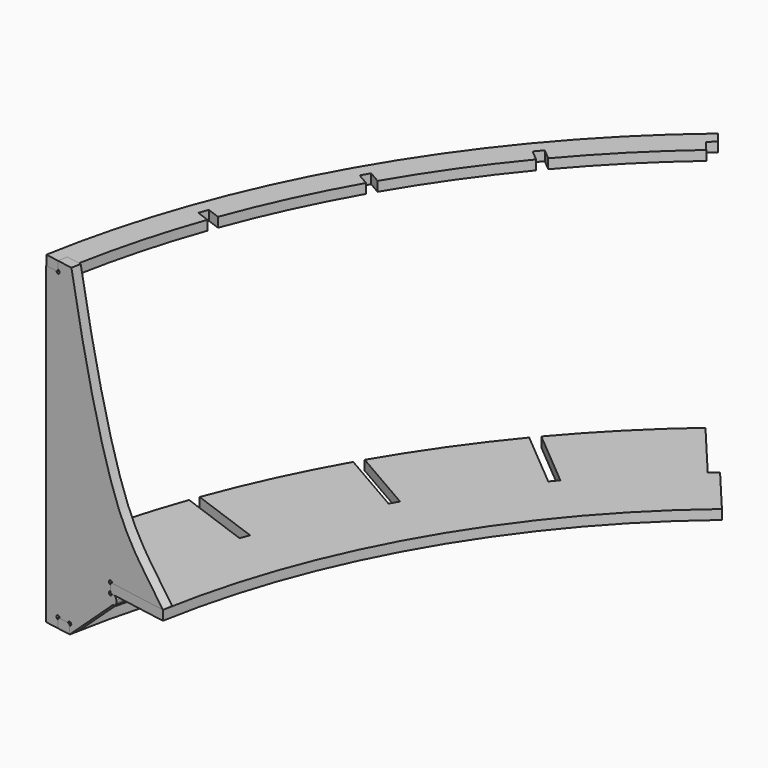
from build123d import *

# Parameters (mm, degrees)
F1_DEPTH = 17.78
F3_DEPTH = 17.78
F5_DEPTH = 17.78
F8_DEPTH = 17.78


with BuildPart() as f1:
    # F0 (on Top) → F1 (new body)
    with BuildSketch(Plane.XY):
        with BuildLine():
            Line((-942.8730052687, 1123.6722913891), (-959.1998105547, 1143.1298202443))
            ThreePointArc((-959.1998105547, 1143.1298202443), (-965.9930441933, 1137.395050574), (-972.7519920849, 1131.6199116288))
            Line((-972.7519920849, 1131.6199116288), (-989.0799370092, 1151.0787986519))
            ThreePointArc((-989.0799370092, 1151.0787986519), (-1076.2792142324, 1069.9927922707), (-1156.8530210759, 982.3200141133))
            Line((-1156.8530210759, 982.3200141133), (-1137.3951527054, 965.9929239401))
            ThreePointArc((-1137.3951527054, 965.9929239401), (-1143.1298202443, 959.1998105547), (-1148.8239164056, 952.3726537414))
            Line((-1148.8239164056, 952.3726537414), (-1168.2817847761, 968.6997439146))
            ThreePointArc((-1168.2817847761, 968.6997439146), (-1243.1861000152, 870.4882786282), (-1309.8559045877, 766.5109468995))
            Line((-1309.8559045877, 766.5109468995), (-1287.8584755041, 753.8107252966))
            ThreePointArc((-1287.8584755041, 753.8107252966), (-1292.3264087973, 746.125), (-1296.7484755041, 738.4127936173))
            Line((-1296.7484755041, 738.4127936173), (-1318.7459045877, 751.1130152202))
            ThreePointArc((-1318.7459045877, 751.1130152202), (-1375.4580129962, 641.3866049308), (-1423.0594792576, 527.4118324374))
            Line((-1423.0594792576, 527.4118324374), (-1399.1908702125, 518.7243692117))
            ThreePointArc((-1399.1908702125, 518.7243692117), (-1402.2563133678, 510.3795588777), (-1405.2719883608, 502.0166344141))
            Line((-1405.2719883608, 502.0166344141), (-1429.140597406, 510.7040976399))
            ThreePointArc((-1429.140597406, 510.7040976399), (-1464.7805470889, 397.088744955), (-1491.4034498948, 281.0289524975))
            Line((-1491.4034498948, 281.0289524975), (-1466.3875869413, 276.6179809131))
            ThreePointArc((-1466.3875869413, 276.6179809131), (-1468.0095300324, 267.8769908634), (-1469.5793694325, 259.1264931235))
            Line((-1469.5793694325, 259.1264931235), (-1444.565252506, 254.7158294107))
            ThreePointArc((-1444.565252506, 254.7158294107), (-1270.3293635412, 733.425), (-942.8730052687, 1123.6722913891))
        make_face()
    extrude(amount=F1_DEPTH)


with BuildPart() as f3:
    # F2 (on face) → F3 (new body)
    with BuildSketch(Plane(origin=(0, 0, 0), x_dir=(0.984807753, -0.1736481777, 0), z_dir=(-0.1736481777, -0.984807753, 0))):
        with BuildLine():
            Line((-1518.3551311493, 0), (-1492.25, 0))
            Line((-1492.25, 0), (-1492.25, 14.351))
            ThreePointArc((-1492.25, 14.351), (-1494.6746691527, 20.2046691527), (-1488.821, 17.78))
            Line((-1488.821, 17.78), (-1470.2938070244, 17.78))
            ThreePointArc((-1470.2938070244, 17.78), (-1464.4415489784, 20.1951790962), (-1466.85, 14.3401489527))
            Line((-1466.85, 14.3401489527), (-1466.85, 0))
            Line((-1466.85, 0), (-1374.1479773797, 83.4850971333))
            ThreePointArc((-1374.1479773797, 83.4850971333), (-1372.5673341992, 84.5284814934), (-1370.7492766555, 85.0592832973))
            ThreePointArc((-1370.7492766555, 85.0592832973), (-1366.8185465998, 87.1734978195), (-1365.25, 91.3520386391))
            Line((-1365.25, 91.3520386391), (-1365.25, 95.25))
            ThreePointArc((-1365.25, 95.25), (-1367.1098719395, 99.7401280605), (-1371.6, 101.6))
            Line((-1371.6, 101.6), (-1374.5770201141, 101.6))
            ThreePointArc((-1374.5770201141, 101.6), (-1380.4069192448, 99.0381939532), (-1377.95, 104.9130660301))
            Line((-1377.95, 104.9130660301), (-1377.95, 116.0374188485))
            ThreePointArc((-1377.95, 116.0374188485), (-1380.3385150421, 121.9228376163), (-1374.5181082663, 119.38))
            Line((-1374.5181082663, 119.38), (-1263.6500000001, 119.38))
            add(Edge.make_bspline(
                [(-1463.0953241153, 596.9), (-1435.2213655624, 463.1560709507), (-1371.53772684, 219.6405486266), (-1300.5032324543, 163.3910187016), (-1263.6500000001, 119.38)],
                knots=[0.0910439939, 0.0910439939, 0.0910439939, 0.0910439939, 0.6287928425, 1, 1, 1, 1], degree=3))
            Line((-1463.0953241153, 596.9), (-1492.25, 596.9))
            Line((-1492.25, 596.9), (-1492.25, 582.7054097958))
            ThreePointArc((-1492.25, 582.7054097958), (-1489.6412751046, 576.9444635359), (-1495.5793714733, 579.12))
            Line((-1495.5793714733, 579.12), (-1518.3551311493, 579.12))
            Line((-1518.3551311493, 579.12), (-1518.3551311493, 0))
        make_face()
    extrude(amount=-F3_DEPTH)


with BuildPart() as f5:
    # F4 (on face) → F5 (new body)
    with BuildSketch(Plane.XY.offset(579.12)):
        with BuildLine():
            ThreePointArc((-1168.2817847761, 968.6997439146), (-1243.1861000152, 870.4882786282), (-1309.8559045877, 766.5109468995))
            ThreePointArc((-1309.8559045877, 766.5109468995), (-1375.4580129962, 641.3866049308), (-1429.140597406, 510.7040976399))
            ThreePointArc((-1429.140597406, 510.7040976399), (-1467.0814981789, 388.5014803077), (-1494.593486359, 263.5371568362))
            Line((-1494.593486359, 263.5371568362), (-1469.5793694325, 259.1264931235))
            Line((-1469.5793694325, 259.1264931235), (-1466.4919048335, 276.636374972))
            Line((-1466.4919048335, 276.636374972), (-1441.3716635128, 272.2069986653))
            ThreePointArc((-1441.3716635128, 272.2069986653), (-1415.7112941773, 383.940690783), (-1381.4033648918, 493.3291659385))
            Line((-1381.4033648918, 493.3291659385), (-1405.2719883608, 502.0166344141))
            ThreePointArc((-1405.2719883608, 502.0166344141), (-1402.2563133678, 510.3795588777), (-1399.1908702125, 518.7243692117))
            Line((-1399.1908702125, 518.7243692117), (-1375.3222467435, 510.0369007361))
            ThreePointArc((-1375.3222467435, 510.0369007361), (-1329.4175774147, 619.9175972343), (-1274.7510331275, 725.7125643397))
            Line((-1274.7510331275, 725.7125643397), (-1296.7484755041, 738.4127936173))
            ThreePointArc((-1296.7484755041, 738.4127936173), (-1292.3264087973, 746.125), (-1287.8584755041, 753.8107252966))
            Line((-1287.8584755041, 753.8107252966), (-1265.8610331275, 741.110496019))
            ThreePointArc((-1265.8610331275, 741.110496019), (-1201.5731761653, 841.3505956615), (-1129.3660362767, 936.0455537017))
            Line((-1129.3660362767, 936.0455537017), (-1148.8239164056, 952.3726537414))
            ThreePointArc((-1148.8239164056, 952.3726537414), (-1143.1298202443, 959.1998105547), (-1137.3951527054, 965.9929239401))
            Line((-1137.3951527054, 965.9929239401), (-1117.9372725764, 949.6658239004))
            ThreePointArc((-1117.9372725764, 949.6658239004), (-1040.3580388533, 1034.0715997906), (-956.4240076884, 1112.1609775645))
            Line((-956.4240076884, 1112.1609775645), (-972.7519920849, 1131.6199116288))
            Line((-972.7519920849, 1131.6199116288), (-959.1998105547, 1143.1298202443))
            Line((-959.1998105547, 1143.1298202443), (-975.5266158408, 1162.5873490995))
            ThreePointArc((-975.5266158408, 1162.5873490995), (-1076.2791066912, 1069.9929004437), (-1168.2817847761, 968.6997439146))
        make_face()
    extrude(amount=F5_DEPTH)


with BuildPart() as f8:
    # F7 (on face) → F8 (new body)
    with BuildSketch(Plane(origin=(0, 0, 119.38), x_dir=(1, 0, 0), z_dir=(0, 0, -1))):
        with BuildLine():
            Line((-1357.0158432632, -239.2785064161), (-1353.9283786643, -256.7883882647))
            Line((-1353.9283786643, -256.7883882647), (-1491.4034498948, -281.0289524975))
            ThreePointArc((-1491.4034498948, -281.0289524975), (-1464.7805470889, -397.088744955), (-1429.140597406, -510.7040976399))
            Line((-1429.140597406, -510.7040976399), (-1297.8630576463, -462.9229807397))
            Line((-1297.8630576463, -462.9229807397), (-1291.781939498, -479.6307155373))
            Line((-1291.781939498, -479.6307155373), (-1423.0594792576, -527.4118324374))
            ThreePointArc((-1423.0594792576, -527.4118324374), (-1375.4580129962, -641.3866049308), (-1318.7459045877, -751.1130152202))
            Line((-1318.7459045877, -751.1130152202), (-1197.7598695127, -681.2616953015))
            Line((-1197.7598695127, -681.2616953015), (-1188.8698695127, -696.6596269808))
            Line((-1188.8698695127, -696.6596269808), (-1309.8559045877, -766.5109468995))
            ThreePointArc((-1309.8559045877, -766.5109468995), (-1243.1861000152, -870.4882786282), (-1168.2817847761, -968.6997439146))
            Line((-1168.2817847761, -968.6997439146), (-1061.2633538396, -878.9006179866))
            Line((-1061.2633538396, -878.9006179866), (-1049.8345901393, -892.5208881852))
            Line((-1049.8345901393, -892.5208881852), (-1156.8530210759, -982.3200141133))
            ThreePointArc((-1156.8530210759, -982.3200141133), (-1076.2792142324, -1069.9927922707), (-989.0799370092, -1151.0787986519))
            Line((-989.0799370092, -1151.0787986519), (-899.2757199376, -1044.0543003268))
            Line((-899.2757199376, -1044.0543003268), (-885.7291867676, -1055.5709403958))
            Line((-885.7291867676, -1055.5709403958), (-812.2585629805, -968.0120605474))
            ThreePointArc((-812.2585629805, -968.0120605474), (-1094.3530014923, -631.825), (-1244.452317094, -219.4305197088))
            Line((-1244.452317094, -219.4305197088), (-1357.0158432632, -239.2785064161))
        make_face()
    extrude(amount=F8_DEPTH)


solid = Compound([f1.part, f3.part, f5.part, f8.part])
